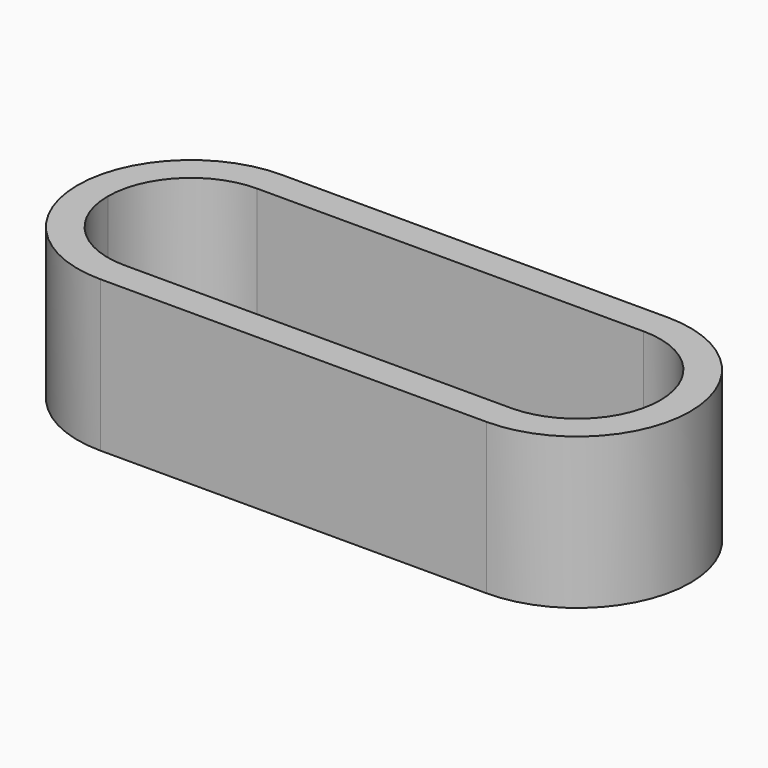
from build123d import *

# Parameters (mm, degrees)
F1_DEPTH = 5


with BuildPart() as f1:
    # F0 (on Top) → F1 (new body)
    with BuildSketch(Plane.XY):
        with BuildLine():
            ThreePointArc((-10.1051355834, 0), (-9.2996792316, 1.9445436483), (-7.3551355834, 2.75))
            Line((-7.3551355834, 2.75), (-4.8056258266, 2.75))
            ThreePointArc((-4.8056258266, 2.75), (-5.9858291896, 3.4910600109), (-7.3551355834, 3.75))
            ThreePointArc((-7.3551355834, 3.75), (-11.1051355834, 0), (-7.3551355834, -3.75))
            ThreePointArc((-7.3551355834, -3.75), (-5.9858291896, -3.4910600109), (-4.8056258266, -2.75))
            Line((-4.8056258266, -2.75), (-7.3551355834, -2.75))
            ThreePointArc((-7.3551355834, -2.75), (-9.2996792316, -1.9445436483), (-10.1051355834, 0))
        make_face()
        with BuildLine():
            ThreePointArc((-7.3551355834, 3.75), (-5.9858291896, 3.4910600109), (-4.8056258266, 2.75))
            Line((-4.8056258266, 2.75), (2.8953546598, 2.75))
            ThreePointArc((2.8953546598, 2.75), (4.0755580229, 3.4910600109), (5.4448644166, 3.75))
            Line((5.4448644166, 3.75), (-7.3551355834, 3.75))
        make_face()
        with BuildLine():
            ThreePointArc((5.4448644166, 3.75), (4.0755580229, 3.4910600109), (2.8953546598, 2.75))
            Line((2.8953546598, 2.75), (5.4448644166, 2.75))
            ThreePointArc((5.4448644166, 2.75), (7.3894080649, 1.9445436483), (8.1948644166, 0))
            ThreePointArc((8.1948644166, 0), (7.3894080649, -1.9445436483), (5.4448644166, -2.75))
            Line((5.4448644166, -2.75), (2.8953546598, -2.75))
            ThreePointArc((2.8953546598, -2.75), (4.0755580229, -3.4910600109), (5.4448644166, -3.75))
            ThreePointArc((5.4448644166, -3.75), (8.0965148461, -2.6516504294), (9.1948644166, 0))
            ThreePointArc((9.1948644166, 0), (8.0965148461, 2.6516504294), (5.4448644166, 3.75))
        make_face()
        with BuildLine():
            Line((2.8953546598, -2.75), (-4.8056258266, -2.75))
            ThreePointArc((-4.8056258266, -2.75), (-5.9858291896, -3.4910600109), (-7.3551355834, -3.75))
            Line((-7.3551355834, -3.75), (5.4448644166, -3.75))
            ThreePointArc((5.4448644166, -3.75), (4.0755580229, -3.4910600109), (2.8953546598, -2.75))
        make_face()
    extrude(amount=F1_DEPTH)


solid = f1.part
